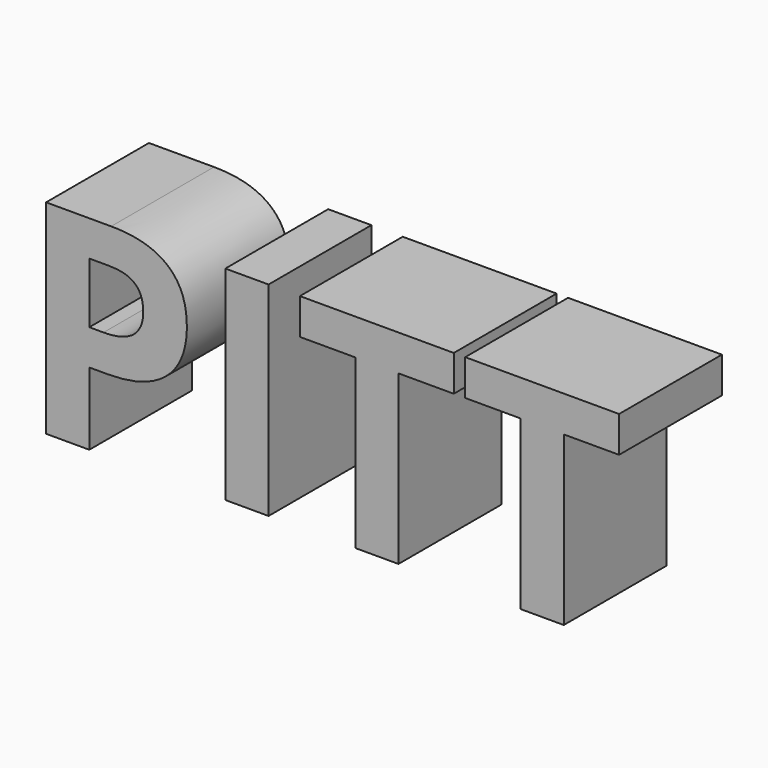
from build123d import *

# Parameters (mm, degrees)
F0_TEXT_SIZE = 56.402064962
F1_DEPTH     = 25.4


# Not quite as in the source:
# - Text() gives the source's letters only with a copy of the font that has no kerning and outlines rounded to 1/6400 em; it was checked with that copy


with BuildPart() as f1:
    # F0 (on Front) → F1 (new body)
    with BuildSketch(Plane.XZ):
        with Locations((-61.1540678226, -20.8529213541)):
            Text('PITT', F0_TEXT_SIZE, font='Open Sans', font_style=FontStyle.BOLD, text_align=(TextAlign.LEFT, TextAlign.BOTTOM))
    extrude(amount=F1_DEPTH)


solid = f1.part
